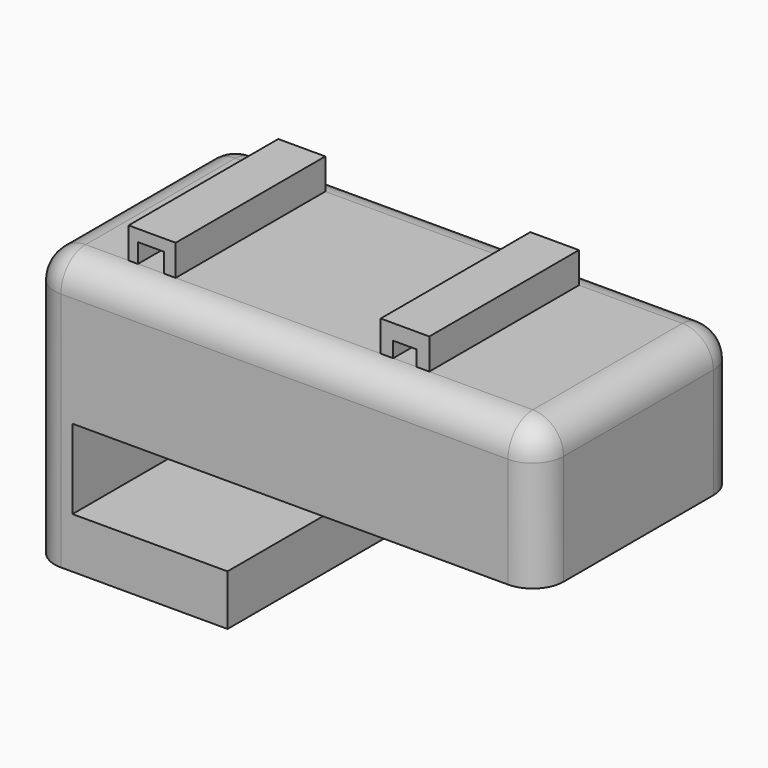
from build123d import *

# Parameters (mm, degrees)
F1_DEPTH    = 40.894
F2_R        = 5.08
F3_T1_DEPTH = 52.2452971888
F3_S5_W     = 5.08
F3_S5_H     = 5.08
F3_T6_DEPTH = 5.08
F4_W        = 7.728997618
F4_H        = 30.734
F4_W_2      = 7.9892426729
F5_DEPTH    = 5.08
F6_W        = 4.2550079525
F6_H        = 3.1596273184
F6_W_2      = 3.8497596979
F6_H_2      = 2.54
F7_DEPTH    = 39.37


# Not quite as in the source:
# - a fillet or chamfer that OpenCascade refuses, or shapes differently, is made with other operations: its cross-section is extruded or revolved along the edge and cut away or added
# - a feature of the source that left no trace in its solid (it failed there, or was rolled back) is left out


with BuildPart() as f1:
    # F0 (on Front) → F1 (new body)
    with BuildSketch(Plane.XZ):
        Polygon((45.526817441, 12.0578445494), (-38.0892679095, 12.0578445494), (-38.0892679095, -11.1563242972), (-38.0892679095, -32.5674526393), (-5.6345071644, -32.5674526393), (-5.6345071644, -24.228380993), (-31.1024785042, -24.228380993), (-31.1024785042, -11.1563242972), (45.526817441, -11.1563242972), align=None)
    extrude(amount=F1_DEPTH)

    # F2
    f2_edges = [f1.edges().sort_by_distance(p)[0] for p in [
        (45.526817, 0, 0.45076),
        (45.526817, -40.894, 0.45076),
        (-38.089268, 0, -10.254804),
        (3.718775, 0, 12.057845),
        (3.718775, -40.894, 12.057845),
        (45.526817, -20.447, 12.057845),
        (-38.089268, -20.447, 12.057845),
    ]]
    fillet(f2_edges, radius=F2_R)

    # F3: fillet of radius 5.08 on 1 edges, made by hand

    # F3_s2 → F3_t1 (cut)
    with BuildSketch(Plane.XY.offset(-45.2674526393)):
        with BuildLine():
            ThreePointArc((-38.0892679095, -35.814), (-36.601370358, -39.4061024484), (-33.0092679095, -40.894))
            Line((-33.0092679095, -40.894), (-38.0892679095, -40.894))
            Line((-38.0892679095, -40.894), (-38.0892679095, -35.814))
        make_face()
    extrude(amount=F3_T1_DEPTH, mode=Mode.SUBTRACT)


with BuildPart() as f3_tool4:
    # F3_s5 → F3_t6 (new body)
    with BuildSketch(Plane.YZ.offset(-33.0092679095)):
        with Locations((-38.354, 9.5178445494)):
            Rectangle(F3_S5_W, F3_S5_H)
    extrude(amount=-F3_T6_DEPTH)

    # F3_s7 → F3_t8 (revolve, cut)
    with BuildSketch(Plane(origin=(-33.0092679095, -35.814, 6.9778445494), x_dir=(0, 0.7071067812, -0.7071067812), z_dir=(0, 0.7071067812, 0.7071067812))):
        with BuildLine():
            ThreePointArc((0, -5.08), (5.08, 0), (0, 5.08))
            Line((0, 5.08), (0, -5.08))
        make_face()
    revolve(axis=Axis((-33.0092679095, -35.814, 6.9778445494), (-1, 0, 0)), mode=Mode.SUBTRACT)


with BuildPart() as f1_1:
    add(f1.part)

    # F3_t3: cut F3_tool4
    add(f3_tool4.part, mode=Mode.SUBTRACT)

    # F4 (on face) → F5 (join)
    with BuildSketch(Plane.XY.offset(12.0578445494)):
        with Locations((-22.0848601311, -20.447)):
            Rectangle(F4_W, F4_H)
        with Locations((19.4605253637, -20.447)):
            Rectangle(F4_W_2, F4_H)
    extrude(amount=F5_DEPTH)

    # F6 (on face) → F7 (cut)
    with BuildSketch(Plane.XZ.offset(35.814)):
        with Locations((-22.2941972315, 13.6376582086)):
            Rectangle(F6_W, F6_H)
        with Locations((19.4453038275, 13.3278445494)):
            Rectangle(F6_W_2, F6_H_2)
    extrude(amount=-F7_DEPTH, mode=Mode.SUBTRACT)


solid = f1_1.part
